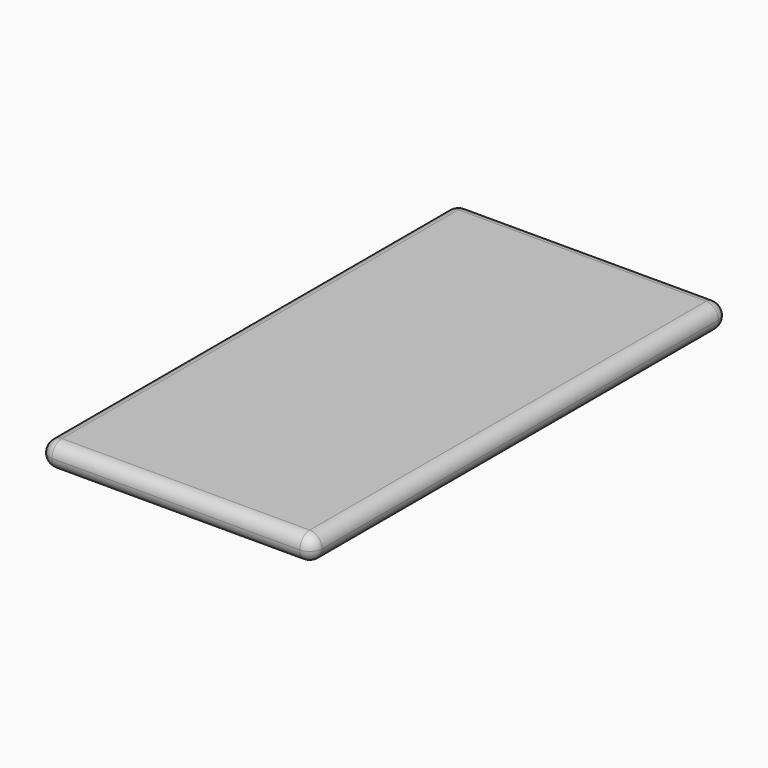
from build123d import *

# Parameters (mm, degrees)
F0_W     = 110
F0_H     = 210
F1_DEPTH = 10
F2_R     = 4.99999


# Not quite as in the source:
# - a fillet or chamfer is up to 0.001 mm smaller than in the source, because OpenCascade refuses the exact size


with BuildPart() as f1:
    # F0 (on Top) → F1 (new body)
    with BuildSketch(Plane.XY):
        Rectangle(F0_W, F0_H)
    extrude(amount=F1_DEPTH)

    # F2 (radius 5 in the source; OpenCascade refuses exactly that, so slightly less here)
    f2_edges = [f1.edges().sort_by_distance(p)[0] for p in [
        (-55, 0, 10),
        (0, -105, 10),
        (0, -105, 0),
        (-55, -105, 5),
        (-55, 0, 0),
        (-55, 105, 5),
        (0, 105, 10),
        (0, 105, 0),
        (55, 105, 5),
        (55, 0, 10),
        (55, 0, 0),
        (55, -105, 5),
    ]]
    fillet(f2_edges, radius=F2_R)


solid = f1.part
